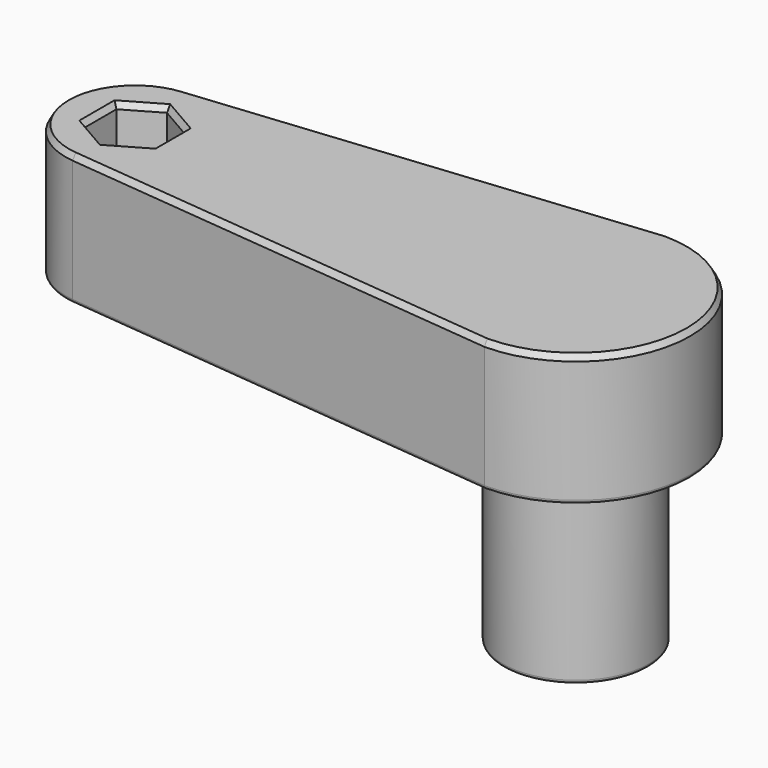
from build123d import *

# Parameters (mm, degrees)
F0_R           = 10.5
F1_DEPTH       = 40
F2_R           = 10.5
F3_DEPTH       = 19
F4_R           = 2
F5_DEPTH       = 7
F6_R           = 3
F7_DEPTH       = 3.5
F9_DEPTH       = 25
F10_R          = 10.5
F10_R_2        = 7.4
F11_DEPTH      = 5
F12_T3_DEPTH   = 68.75
F12_T5_DEPTH   = 68.75
F12_T8_ANGLE   = 168.5216590455
F12_T10_ANGLE  = 188.6951396909
F13_T1_DEPTH   = 68.808819375
F13_T3_DEPTH   = 68.808819375
F13_T6_ANGLE   = 195.5850430697
F13_T8_ANGLE   = 168.5216590455
F13_T12_DEPTH  = 10.2544666625
F13_T18_DEPTH  = 10.2544666625
F13_T24_DEPTH  = 10.2544666625
F13_T30_DEPTH  = 10.2544666625
F13_T36_DEPTH  = 10.2544666625
F13_T42_DEPTH  = 10.2544666625
F13_T49_DEPTH  = 10.2544666625
F13_T53_DEPTH  = 10.2544666625
F13_T60_DEPTH  = 10.2544666625
F13_T64_DEPTH  = 10.2544666625
F13_T71_DEPTH  = 10.2544666625
F13_T75_DEPTH  = 10.2544666625
F13_T82_DEPTH  = 10.2544666625
F13_T86_DEPTH  = 10.2544666625
F13_T93_DEPTH  = 10.2544666625
F13_T97_DEPTH  = 10.2544666625
F13_T104_DEPTH = 10.2544666625
F13_T108_DEPTH = 10.2544666625


# Not quite as in the source:
# - a fillet or chamfer that OpenCascade refuses, or shapes differently, is made with other operations: its cross-section is extruded or revolved along the edge and cut away or added


with BuildPart() as f1:
    # F0 (on Top) → F1 (new body)
    with BuildSketch(Plane.XY):
        Circle(F0_R)
    extrude(amount=F1_DEPTH)

    # F2 (on face) → F3 (join)
    with BuildSketch(Plane.XY.offset(40)):
        with BuildLine():
            Line((-64.6741834119, -10), (0, -16.5))
            ThreePointArc((0, -16.5), (16.5, 0), (0, 16.5))
            Line((0, 16.5), (-64.6741834119, 10))
            ThreePointArc((-64.6741834119, 10), (-73.7195237493, 0), (-64.6741834119, -10))
        make_face()
        Polygon((-63.6691455967, 5.7735026919), (-58.6691455967, 2.8867513459), (-58.6691455967, -2.8867513459), (-63.6691455967, -5.7735026919), (-68.6691455967, -2.8867513459), (-68.6691455967, 2.8867513459), align=None, mode=Mode.SUBTRACT)
        Circle(F2_R, mode=Mode.SUBTRACT)
    extrude(amount=-F3_DEPTH)

    # F4 (on face) → F5 (join)
    with BuildSketch(Plane(origin=(0, 0, 21), x_dir=(1, 0, 0), z_dir=(0, 0, -1))):
        Polygon((-58.6691455967, 2.8867513459), (-63.6691455967, 5.7735026919), (-68.6691455967, 2.8867513459), (-68.6691455967, -2.8867513459), (-63.6691455967, -5.7735026919), (-58.6691455967, -2.8867513459), align=None)
        with Locations((-63.6691455967, 0)):
            Circle(F4_R, mode=Mode.SUBTRACT)
    extrude(amount=-F5_DEPTH)

    # F6 (on face) → F7 (cut)
    with BuildSketch(Plane(origin=(0, 0, 21), x_dir=(1, 0, 0), z_dir=(0, 0, -1))):
        with Locations((-63.6691455967, 0)):
            Circle(F6_R)
    extrude(amount=-F7_DEPTH, mode=Mode.SUBTRACT)

    # F8 (on face) → F9 (cut)
    with BuildSketch(Plane(origin=(0, 0, 0), x_dir=(1, 0, 0), z_dir=(0, 0, -1))):
        with BuildLine():
            Line((4.5, 5.5), (-4.5, 5.5))
            ThreePointArc((-4.5, 5.5), (-5.2071067812, 5.2071067812), (-5.5, 4.5))
            Line((-5.5, 4.5), (-5.5, -4.5))
            ThreePointArc((-5.5, -4.5), (-5.2071067812, -5.2071067812), (-4.5, -5.5))
            Line((-4.5, -5.5), (4.5, -5.5))
            ThreePointArc((4.5, -5.5), (5.2071067812, -5.2071067812), (5.5, -4.5))
            Line((5.5, -4.5), (5.5, 4.5))
            ThreePointArc((5.5, 4.5), (5.2071067812, 5.2071067812), (4.5, 5.5))
        make_face()
    extrude(amount=-F9_DEPTH, mode=Mode.SUBTRACT)

    # F10 (on face) → F11 (join)
    with BuildSketch(Plane(origin=(0, 0, 0), x_dir=(1, 0, 0), z_dir=(0, 0, -1))):
        Circle(F10_R)
        Circle(F10_R_2, mode=Mode.SUBTRACT)
    extrude(amount=F11_DEPTH)

    # F12: fillet of radius 0.5 on 9 edges, made by hand

    # F12_s1 → F12_t2 (revolve)
    with BuildSketch(Plane.XZ):
        with BuildLine():
            ThreePointArc((10.5, 20.5), (10.6464466094, 20.8535533906), (11, 21))
            Line((11, 21), (10.5, 21))
            Line((10.5, 21), (10.5, 20.5))
        make_face()
    revolve(axis=Axis((0, 0, 21), (0, 0, 1)))

    # F12_s4 → F12_t3 (cut)
    with BuildSketch(Plane(origin=(-63.0324541407, 6.335, 0), x_dir=(0, 0, 1), z_dir=(0.9949874371, -0.1, 0))):
        with BuildLine():
            ThreePointArc((21, 15.9172927123), (21.1464466094, 16.2708461029), (21.5, 16.4172927123))
            Line((21.5, 16.4172927123), (21, 16.4172927123))
            Line((21, 16.4172927123), (21, 15.9172927123))
        make_face()
    extrude(amount=F12_T3_DEPTH, mode=Mode.SUBTRACT)

    # F12_s6 → F12_t5 (cut)
    with BuildSketch(Plane(origin=(5.3729321604, 0.54, 0), x_dir=(0, 0, 1), z_dir=(-0.9949874371, -0.1, 0))):
        with BuildLine():
            ThreePointArc((21, 15.9172927123), (21.1464466094, 16.2708461029), (21.5, 16.4172927123))
            Line((21.5, 16.4172927123), (21, 16.4172927123))
            Line((21, 16.4172927123), (21, 15.9172927123))
        make_face()
    extrude(amount=F12_T5_DEPTH, mode=Mode.SUBTRACT)

    # F12_s7 → F12_t8 (revolve, cut)
    with BuildSketch(Plane(origin=(-63.0324541407, -6.335, 0), x_dir=(0, 0, 1), z_dir=(0.9949874371, 0.1, 0))):
        with BuildLine():
            ThreePointArc((21, -15.9172927123), (21.1464466094, -16.2708461029), (21.5, -16.4172927123))
            Line((21.5, -16.4172927123), (21, -16.4172927123))
            Line((21, -16.4172927123), (21, -15.9172927123))
        make_face()
    revolve(axis=Axis((-63.6691455967, 0, 21), (0, 0, 1)), revolution_arc=F12_T8_ANGLE, mode=Mode.SUBTRACT)

    # F12_s9 → F12_t10 (revolve, cut)
    with BuildSketch(Plane(origin=(0, 0, 0), x_dir=(0, 0, 1), z_dir=(-0.9971225387, 0.0758066143, 0))):
        with BuildLine():
            ThreePointArc((21, -16), (21.1464466094, -16.3535533906), (21.5, -16.5))
            Line((21.5, -16.5), (21, -16.5))
            Line((21, -16.5), (21, -16))
        make_face()
    revolve(axis=Axis((0, 0, 21), (0, 0, 1)), revolution_arc=F12_T10_ANGLE, mode=Mode.SUBTRACT)

    # F12_s11 → F12_t12 (revolve, cut)
    with BuildSketch(Plane.XZ):
        with BuildLine():
            ThreePointArc((-60.1691455967, 21), (-60.5226989873, 21.1464466094), (-60.6691455967, 21.5))
            Line((-60.6691455967, 21.5), (-60.6691455967, 21))
            Line((-60.6691455967, 21), (-60.1691455967, 21))
        make_face()
    revolve(axis=Axis((-63.6691455967, 0, 21), (0, 0, -1)), mode=Mode.SUBTRACT)

    # F12_s13 → F12_t14 (revolve, cut)
    with BuildSketch(Plane.XZ):
        with BuildLine():
            ThreePointArc((-61.1691455967, 24.5), (-61.5226989873, 24.6464466094), (-61.6691455967, 25))
            Line((-61.6691455967, 25), (-61.6691455967, 24.5))
            Line((-61.6691455967, 24.5), (-61.1691455967, 24.5))
        make_face()
    revolve(axis=Axis((-63.6691455967, 0, 24.5), (0, 0, -1)), mode=Mode.SUBTRACT)

    # F12_s15 → F12_t16 (revolve, cut)
    with BuildSketch(Plane.XZ):
        with BuildLine():
            ThreePointArc((10.5, -4.5), (10.3535533906, -4.8535533906), (10, -5))
            Line((10, -5), (10.5, -5))
            Line((10.5, -5), (10.5, -4.5))
        make_face()
    revolve(axis=Axis((0, 0, -5), (0, 0, -1)), mode=Mode.SUBTRACT)

    # F12_s17 → F12_t18 (revolve, cut)
    with BuildSketch(Plane.XZ):
        with BuildLine():
            ThreePointArc((7.9, -5), (7.5464466094, -4.8535533906), (7.4, -4.5))
            Line((7.4, -4.5), (7.4, -5))
            Line((7.4, -5), (7.9, -5))
        make_face()
    revolve(axis=Axis((0, 0, -5), (0, 0, -1)), mode=Mode.SUBTRACT)

    # F13: chamfer of 0.5 x 0.8660254038 on 10 edges, made by hand

    # F13_s2 → F13_t1 (cut)
    with BuildSketch(Plane(origin=(-63.0324541407, 6.335, 0), x_dir=(0, 0, 1), z_dir=(0.9949874371, -0.1, 0))):
        Polygon((39.1339745962, 16.4172927123), (40, 15.9172927123), (40, 16.4172927123), align=None)
    extrude(amount=F13_T1_DEPTH, mode=Mode.SUBTRACT)

    # F13_s4 → F13_t3 (cut)
    with BuildSketch(Plane(origin=(5.4314566996, 0.5458819375, 0), x_dir=(0, 0, 1), z_dir=(-0.9949874371, -0.1, 0))):
        Polygon((39.1339745962, 16.4172927123), (40, 15.9172927123), (40, 16.4172927123), align=None)
    extrude(amount=F13_T3_DEPTH, mode=Mode.SUBTRACT)

    # F13_s5 → F13_t6 (revolve, cut)
    with BuildSketch(Plane(origin=(0, 0, 0), x_dir=(0, 0, 1), z_dir=(-0.9907655461, 0.1355862551, 0))):
        Polygon((39.1339745962, -16.5), (40, -16), (40, -16.5), align=None)
    revolve(axis=Axis((0, 0, 40), (0, 0, 1)), revolution_arc=F13_T6_ANGLE, mode=Mode.SUBTRACT)

    # F13_s7 → F13_t8 (revolve, cut)
    with BuildSketch(Plane(origin=(-63.0324541407, -6.335, 0), x_dir=(0, 0, 1), z_dir=(0.9949874371, 0.1, 0))):
        Polygon((39.1339745962, -16.4172927123), (40, -15.9172927123), (40, -16.4172927123), align=None)
    revolve(axis=Axis((-63.6691455967, 0, 40), (0, 0, 1)), revolution_arc=F13_T8_ANGLE, mode=Mode.SUBTRACT)


with BuildPart() as f13_tool10:
    # F13_s11 → F13_t12 (new body)
    with BuildSketch(Plane(origin=(-52.1921735135, -30.1331654276, 0), x_dir=(0, 0, 1), z_dir=(0.8660254038, 0.5, 0))):
        Polygon((40, -37.3345727983), (39.1339745962, -36.8345727983), (40, -36.8345727983), align=None)
    extrude(amount=F13_T12_DEPTH)

    split(bisect_by=Plane(origin=(-13.4172863992, -23.2394217431, 0), x_dir=(0, 0, 1), z_dir=(-0.5, -0.8660254038, 0)), keep=Keep.TOP)

    split(bisect_by=Plane.YZ.offset(-68.6691455967), keep=Keep.TOP)


with BuildPart() as f1_1:
    add(f1.part)

    # F13_t9: cut F13_tool10
    add(f13_tool10.part, mode=Mode.SUBTRACT)


with BuildPart() as f13_tool16:
    # F13_s17 → F13_t18 (new body)
    with BuildSketch(Plane(origin=(-52.1921735135, 30.1331654276, 0), x_dir=(0, 0, 1), z_dir=(0.8660254038, -0.5, 0))):
        Polygon((40, 26.3345727983), (39.1339745962, 26.8345727983), (40, 26.8345727983), align=None)
    extrude(amount=F13_T18_DEPTH)

    split(bisect_by=Plane(origin=(-18.4172863992, 31.8996757809, 0), x_dir=(0, 0, 1), z_dir=(0.5, -0.8660254038, 0)), keep=Keep.TOP)

    split(bisect_by=Plane.YZ.offset(-58.6691455967), keep=Keep.BOTTOM)


with BuildPart() as f1_2:
    add(f1_1.part)

    # F13_t15: cut F13_tool16
    add(f13_tool16.part, mode=Mode.SUBTRACT)


with BuildPart() as f13_tool22:
    # F13_s23 → F13_t24 (new body)
    with BuildSketch(Plane.XZ.offset(-5.1272333312)):
        Polygon((-58.1691455967, 40), (-58.6691455967, 39.1339745962), (-58.6691455967, 40), align=None)
    extrude(amount=F13_T24_DEPTH)

    split(bisect_by=Plane(origin=(-13.4172863992, -23.2394217431, 0), x_dir=(0, 0, 1), z_dir=(-0.5, -0.8660254038, 0)), keep=Keep.TOP)

    split(bisect_by=Plane(origin=(-13.4172863992, 23.2394217431, 0), x_dir=(0, 0, 1), z_dir=(-0.5, 0.8660254038, 0)), keep=Keep.TOP)


with BuildPart() as f1_3:
    add(f1_2.part)

    # F13_t21: cut F13_tool22
    add(f13_tool22.part, mode=Mode.SUBTRACT)


with BuildPart() as f13_tool28:
    # F13_s29 → F13_t30 (new body)
    with BuildSketch(Plane(origin=(-43.3115448815, -25.0059320964, 0), x_dir=(0, 0, 1), z_dir=(-0.8660254038, -0.5, 0))):
        Polygon((40, 26.3345727983), (39.1339745962, 26.8345727983), (40, 26.8345727983), align=None)
    extrude(amount=F13_T30_DEPTH)

    split(bisect_by=Plane.YZ.offset(-58.6691455967), keep=Keep.BOTTOM)

    split(bisect_by=Plane(origin=(-18.4172863992, -31.8996757809, 0), x_dir=(0, 0, 1), z_dir=(0.5, 0.8660254038, 0)), keep=Keep.TOP)


with BuildPart() as f1_4:
    add(f1_3.part)

    # F13_t27: cut F13_tool28
    add(f13_tool28.part, mode=Mode.SUBTRACT)


with BuildPart() as f13_tool34:
    # F13_s35 → F13_t36 (new body)
    with BuildSketch(Plane(origin=(-43.3115448815, 25.0059320964, 0), x_dir=(0, 0, 1), z_dir=(-0.8660254038, 0.5, 0))):
        Polygon((40, -37.3345727983), (39.1339745962, -36.8345727983), (40, -36.8345727983), align=None)
    extrude(amount=F13_T36_DEPTH)

    split(bisect_by=Plane(origin=(-13.4172863992, 23.2394217431, 0), x_dir=(0, 0, 1), z_dir=(-0.5, 0.8660254038, 0)), keep=Keep.TOP)

    split(bisect_by=Plane.YZ.offset(-68.6691455967), keep=Keep.TOP)


with BuildPart() as f1_5:
    add(f1_4.part)

    # F13_t33: cut F13_tool34
    add(f13_tool34.part, mode=Mode.SUBTRACT)


with BuildPart() as f13_tool40:
    # F13_s41 → F13_t42 (new body)
    with BuildSketch(Plane.XZ.offset(5.1272333312)):
        Polygon((-69.1691455967, 40), (-68.6691455967, 39.1339745962), (-68.6691455967, 40), align=None)
    extrude(amount=-F13_T42_DEPTH)

    split(bisect_by=Plane(origin=(-18.4172863992, 31.8996757809, 0), x_dir=(0, 0, 1), z_dir=(0.5, -0.8660254038, 0)), keep=Keep.TOP)

    split(bisect_by=Plane(origin=(-18.4172863992, -31.8996757809, 0), x_dir=(0, 0, 1), z_dir=(0.5, 0.8660254038, 0)), keep=Keep.TOP)


with BuildPart() as f1_6:
    add(f1_5.part)

    # F13_t39: cut F13_tool40
    add(f13_tool40.part, mode=Mode.SUBTRACT)


with BuildPart() as f13_tool47:
    # F13_s48 → F13_t49 (new body)
    with BuildSketch(Plane(origin=(-52.1921735135, -30.1331654276, 0), x_dir=(0, 0, 1), z_dir=(0.8660254038, 0.5, 0))):
        Polygon((40, -37.3345727983), (39.1339745962, -36.8345727983), (40, -36.8345727983), align=None)
    extrude(amount=F13_T49_DEPTH)

    split(bisect_by=Plane.YZ.offset(-68.6691455967), keep=Keep.BOTTOM)


with BuildPart() as f13_tool51:
    # F13_s52 → F13_t53 (new body)
    with BuildSketch(Plane.XZ.offset(5.1272333312)):
        Polygon((-69.1691455967, 40), (-68.6691455967, 39.1339745962), (-68.6691455967, 40), align=None)
    extrude(amount=-F13_T53_DEPTH)

    split(bisect_by=Plane(origin=(-18.4172863992, 31.8996757809, 0), x_dir=(0, 0, 1), z_dir=(-0.5, 0.8660254038, 0)), keep=Keep.TOP)


with BuildPart() as f13_tool47_1:
    add(f13_tool47.part)

    # F13_t55: intersect F13_tool51
    add(f13_tool51.part, mode=Mode.INTERSECT)


with BuildPart() as f1_7:
    add(f1_6.part)

    # F13_t45: cut F13_tool47
    add(f13_tool47_1.part, mode=Mode.SUBTRACT)


with BuildPart() as f13_tool58:
    # F13_s59 → F13_t60 (new body)
    with BuildSketch(Plane(origin=(-52.1921735135, -30.1331654276, 0), x_dir=(0, 0, 1), z_dir=(0.8660254038, 0.5, 0))):
        Polygon((40, -37.3345727983), (39.1339745962, -36.8345727983), (40, -36.8345727983), align=None)
    extrude(amount=F13_T60_DEPTH)

    split(bisect_by=Plane(origin=(-13.4172863992, -23.2394217431, 0), x_dir=(0, 0, 1), z_dir=(0.5, 0.8660254038, 0)), keep=Keep.TOP)


with BuildPart() as f13_tool62:
    # F13_s63 → F13_t64 (new body)
    with BuildSketch(Plane(origin=(-52.1921735135, 30.1331654276, 0), x_dir=(0, 0, 1), z_dir=(0.8660254038, -0.5, 0))):
        Polygon((40, 26.3345727983), (39.1339745962, 26.8345727983), (40, 26.8345727983), align=None)
    extrude(amount=F13_T64_DEPTH)

    split(bisect_by=Plane(origin=(-18.4172863992, 31.8996757809, 0), x_dir=(0, 0, 1), z_dir=(-0.5, 0.8660254038, 0)), keep=Keep.TOP)


with BuildPart() as f13_tool58_1:
    add(f13_tool58.part)

    # F13_t66: intersect F13_tool62
    add(f13_tool62.part, mode=Mode.INTERSECT)


with BuildPart() as f1_8:
    add(f1_7.part)

    # F13_t56: cut F13_tool58
    add(f13_tool58_1.part, mode=Mode.SUBTRACT)


with BuildPart() as f13_tool69:
    # F13_s70 → F13_t71 (new body)
    with BuildSketch(Plane(origin=(-52.1921735135, 30.1331654276, 0), x_dir=(0, 0, 1), z_dir=(0.8660254038, -0.5, 0))):
        Polygon((40, 26.3345727983), (39.1339745962, 26.8345727983), (40, 26.8345727983), align=None)
    extrude(amount=F13_T71_DEPTH)

    split(bisect_by=Plane.YZ.offset(-58.6691455967), keep=Keep.TOP)


with BuildPart() as f13_tool73:
    # F13_s74 → F13_t75 (new body)
    with BuildSketch(Plane.XZ.offset(-5.1272333312)):
        Polygon((-58.1691455967, 40), (-58.6691455967, 39.1339745962), (-58.6691455967, 40), align=None)
    extrude(amount=F13_T75_DEPTH)

    split(bisect_by=Plane(origin=(-13.4172863992, -23.2394217431, 0), x_dir=(0, 0, 1), z_dir=(0.5, 0.8660254038, 0)), keep=Keep.TOP)


with BuildPart() as f13_tool69_1:
    add(f13_tool69.part)

    # F13_t77: intersect F13_tool73
    add(f13_tool73.part, mode=Mode.INTERSECT)


with BuildPart() as f1_9:
    add(f1_8.part)

    # F13_t67: cut F13_tool69
    add(f13_tool69_1.part, mode=Mode.SUBTRACT)


with BuildPart() as f13_tool80:
    # F13_s81 → F13_t82 (new body)
    with BuildSketch(Plane.XZ.offset(-5.1272333312)):
        Polygon((-58.1691455967, 40), (-58.6691455967, 39.1339745962), (-58.6691455967, 40), align=None)
    extrude(amount=F13_T82_DEPTH)

    split(bisect_by=Plane(origin=(-13.4172863992, 23.2394217431, 0), x_dir=(0, 0, 1), z_dir=(0.5, -0.8660254038, 0)), keep=Keep.TOP)


with BuildPart() as f13_tool84:
    # F13_s85 → F13_t86 (new body)
    with BuildSketch(Plane(origin=(-43.3115448815, -25.0059320964, 0), x_dir=(0, 0, 1), z_dir=(-0.8660254038, -0.5, 0))):
        Polygon((40, 26.3345727983), (39.1339745962, 26.8345727983), (40, 26.8345727983), align=None)
    extrude(amount=F13_T86_DEPTH)

    split(bisect_by=Plane.YZ.offset(-58.6691455967), keep=Keep.TOP)


with BuildPart() as f13_tool80_1:
    add(f13_tool80.part)

    # F13_t88: intersect F13_tool84
    add(f13_tool84.part, mode=Mode.INTERSECT)


with BuildPart() as f1_10:
    add(f1_9.part)

    # F13_t78: cut F13_tool80
    add(f13_tool80_1.part, mode=Mode.SUBTRACT)


with BuildPart() as f13_tool91:
    # F13_s92 → F13_t93 (new body)
    with BuildSketch(Plane(origin=(-43.3115448815, -25.0059320964, 0), x_dir=(0, 0, 1), z_dir=(-0.8660254038, -0.5, 0))):
        Polygon((40, 26.3345727983), (39.1339745962, 26.8345727983), (40, 26.8345727983), align=None)
    extrude(amount=F13_T93_DEPTH)

    split(bisect_by=Plane(origin=(-18.4172863992, -31.8996757809, 0), x_dir=(0, 0, 1), z_dir=(-0.5, -0.8660254038, 0)), keep=Keep.TOP)


with BuildPart() as f13_tool95:
    # F13_s96 → F13_t97 (new body)
    with BuildSketch(Plane(origin=(-43.3115448815, 25.0059320964, 0), x_dir=(0, 0, 1), z_dir=(-0.8660254038, 0.5, 0))):
        Polygon((40, -37.3345727983), (39.1339745962, -36.8345727983), (40, -36.8345727983), align=None)
    extrude(amount=F13_T97_DEPTH)

    split(bisect_by=Plane(origin=(-13.4172863992, 23.2394217431, 0), x_dir=(0, 0, 1), z_dir=(0.5, -0.8660254038, 0)), keep=Keep.TOP)


with BuildPart() as f13_tool91_1:
    add(f13_tool91.part)

    # F13_t99: intersect F13_tool95
    add(f13_tool95.part, mode=Mode.INTERSECT)


with BuildPart() as f1_11:
    add(f1_10.part)

    # F13_t89: cut F13_tool91
    add(f13_tool91_1.part, mode=Mode.SUBTRACT)


with BuildPart() as f13_tool102:
    # F13_s103 → F13_t104 (new body)
    with BuildSketch(Plane(origin=(-43.3115448815, 25.0059320964, 0), x_dir=(0, 0, 1), z_dir=(-0.8660254038, 0.5, 0))):
        Polygon((40, -37.3345727983), (39.1339745962, -36.8345727983), (40, -36.8345727983), align=None)
    extrude(amount=F13_T104_DEPTH)

    split(bisect_by=Plane.YZ.offset(-68.6691455967), keep=Keep.BOTTOM)


with BuildPart() as f13_tool106:
    # F13_s107 → F13_t108 (new body)
    with BuildSketch(Plane.XZ.offset(5.1272333312)):
        Polygon((-69.1691455967, 40), (-68.6691455967, 39.1339745962), (-68.6691455967, 40), align=None)
    extrude(amount=-F13_T108_DEPTH)

    split(bisect_by=Plane(origin=(-18.4172863992, -31.8996757809, 0), x_dir=(0, 0, 1), z_dir=(-0.5, -0.8660254038, 0)), keep=Keep.TOP)


with BuildPart() as f13_tool102_1:
    add(f13_tool102.part)

    # F13_t110: intersect F13_tool106
    add(f13_tool106.part, mode=Mode.INTERSECT)


with BuildPart() as f1_12:
    add(f1_11.part)

    # F13_t100: cut F13_tool102
    add(f13_tool102_1.part, mode=Mode.SUBTRACT)


solid = f1_12.part
